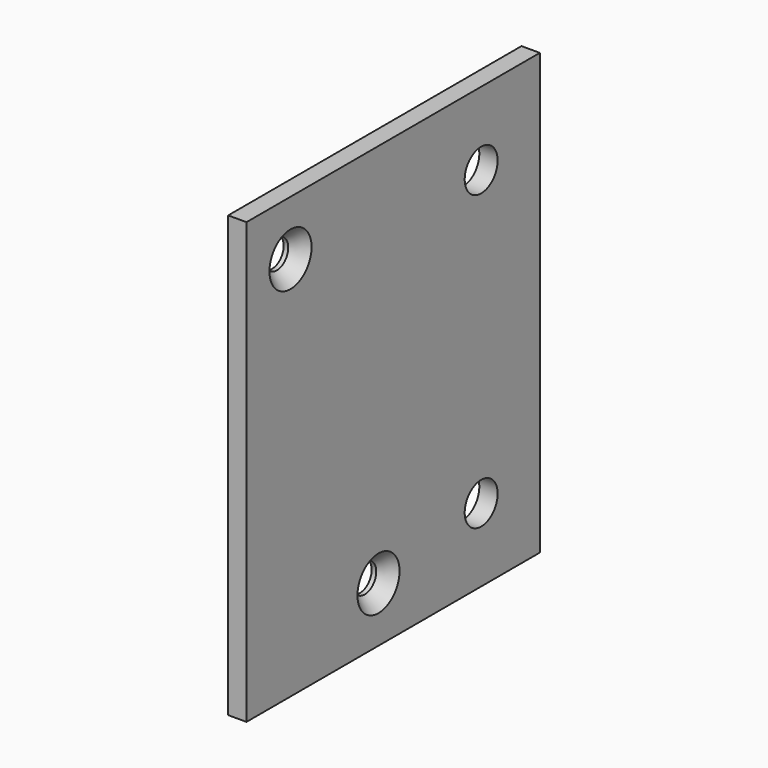
from build123d import *

# Parameters (mm, degrees)
F0_W           = 63.5
F0_H           = 76.2
F1_DEPTH       = 3.175
F3_D           = 4.9784
F3_CSINK_D     = 9.1186
F3_CSINK_ANGLE = 82
F5_D           = 7.1374


# Not quite as in the source:
# - a feature names something its author has since deleted; it is built from what else it names


with BuildPart() as f1:
    # F0 (on Right) → F1 (new body)
    with BuildSketch(Plane.YZ):
        Rectangle(F0_W, F0_H)
    extrude(amount=F1_DEPTH)

    # F3 (through all)
    with Locations(Plane.YZ.offset(3.175)):
        with Locations((-22.225, 28.575), (-3.175, -28.575)):
            CounterSinkHole(F3_D / 2, F3_CSINK_D / 2, counter_sink_angle=F3_CSINK_ANGLE)

    # F5 (through all)
    with Locations(Plane.YZ.offset(3.175)):
        with Locations((19.05, 25.4), (19.05, -25.4)):
            Hole(F5_D / 2)


solid = f1.part
